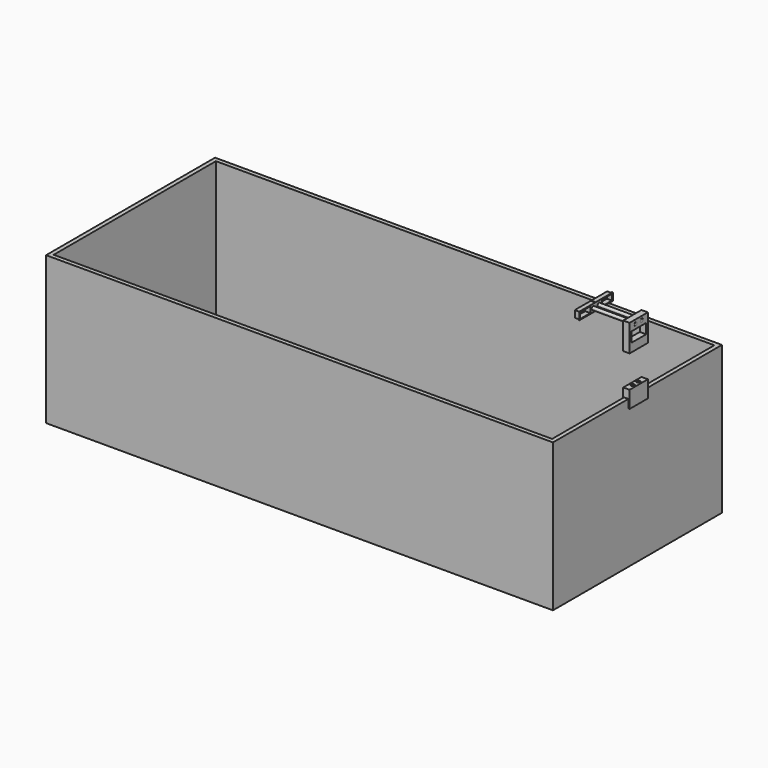
from build123d import *

# Parameters (mm, degrees)
F0_W          = 1.5
F0_H          = 1
F0_H_2        = 16
F0_R          = 4.25
F0_W_2        = 30
F0_H_3        = 14
F1_DEPTH      = 2
F2_DEPTH      = 10
F2_DEPTH_BACK = 2
F5_W          = 1200
F5_H          = 500
F5_W_2        = 1180
F5_H_2        = 480
F6_DEPTH      = 350
F8_W          = 10
F8_H          = 2
F8_W_2        = 1
F8_H_2        = 50
F8_R          = 4.25
F9_DEPTH      = 10
F8_W_3        = 11
F10_DEPTH     = 20
F12_DEPTH     = 15
F13_DEPTH     = 20
F14_W         = 54
F14_H         = 63.75
F14_R         = 4.25
F14_W_2       = 44
F14_H_2       = 23.75
F15_DEPTH     = 15
F16_W         = 110
F16_H         = 4
F19_R         = 4.25
F20_DEPTH     = 15


# Not quite as in the source:
# - a feature names something its author has since deleted; it is built from what else it names
# - the program builds the solid bodies; features that only make, move or delete a surface that nothing else refers to are left out


with BuildPart() as f1:
    # F0 (on Right) → F1 (new body)
    with BuildSketch(Plane.YZ):
        Polygon((-0.75, 9), (-49.5, 9), (-49.5, -9), (-0.75, -9), (-0.75, -8), (-13, -8), (-16, -8), (-48, -8), (-48, 8), (-16, 8), (-13, 8), (-0.75, 8), align=None)
        with Locations((0, 8.5)):
            Rectangle(F0_W, F0_H)
        Polygon((49.5, 9), (0.75, 9), (0.75, 8), (13, 8), (16, 8), (48, 8), (48, -8), (16, -8), (13, -8), (0.75, -8), (0.75, -9), (49.5, -9), align=None)
        with Locations((0, -8.5)):
            Rectangle(F0_W, F0_H)
        Rectangle(F0_W, F0_H_2)
        Polygon((13, 8), (0.75, 8), (0.75, -8), (13, -8), (16, -8), (48, -8), (48, 8), (16, 8), align=None)
        with Locations((8.75, 0)):
            Circle(F0_R, mode=Mode.SUBTRACT)
        with Locations((32, 0)):
            Rectangle(F0_W_2, F0_H_3, mode=Mode.SUBTRACT)
    extrude(amount=F1_DEPTH)

    # F0 (on Right) → F2 (join, two sides)
    with BuildSketch(Plane.YZ) as f2_sk:
        Polygon((-0.75, -8), (-0.75, 8), (-13, 8), (-16, 8), (-48, 8), (-48, -8), (-16, -8), (-13, -8), align=None)
        with Locations((-32, 0)):
            Rectangle(F0_W_2, F0_H_3, mode=Mode.SUBTRACT)
        with Locations((-8.75, 0)):
            Circle(F0_R, mode=Mode.SUBTRACT)
        Polygon((13, 8), (0.75, 8), (0.75, -8), (13, -8), (16, -8), (48, -8), (48, 8), (16, 8), align=None)
        with Locations((8.75, 0)):
            Circle(F0_R, mode=Mode.SUBTRACT)
        with Locations((32, 0)):
            Rectangle(F0_W_2, F0_H_3, mode=Mode.SUBTRACT)
    extrude(amount=-F2_DEPTH)
    extrude(f2_sk.sketch, amount=F2_DEPTH_BACK)


with BuildPart() as f6:
    # F5 (on offset) → F6 (new body)
    with BuildSketch(Plane.XY.offset(-500)):
        with Locations((-500, 0)):
            Rectangle(F5_W, F5_H)
        with Locations((-500, 0)):
            Rectangle(F5_W_2, F5_H_2, mode=Mode.SUBTRACT)
    extrude(amount=F6_DEPTH)


with BuildPart() as f9:
    # F8 (on face) → F9 (new body)
    with BuildSketch(Plane.XY.offset(-150)):
        Polygon((101, 27), (101, 25), (101, -25), (101, -27), (103, -27), (103, 27), align=None)
        Polygon((90, -25), (90, 25), (90, 27), (88, 27), (88, -27), (90, -27), align=None)
        with Locations((95, 26)):
            Rectangle(F8_W, F8_H)
        with Locations((100.5, 26)):
            Rectangle(F8_W_2, F8_H)
        with Locations((100.5, -26)):
            Rectangle(F8_W_2, F8_H)
        with Locations((95, -26)):
            Rectangle(F8_W, F8_H)
        with Locations((100.5, 0)):
            Rectangle(F8_W_2, F8_H_2)
        with Locations((95, 0)):
            Rectangle(F8_W, F8_H_2)
        with Locations((95.5, -8.75)):
            Circle(F8_R, mode=Mode.SUBTRACT)
        with Locations((95.5, 8.75)):
            Circle(F8_R, mode=Mode.SUBTRACT)
        with Locations((95.5, 8.75)):
            Circle(F8_R)
        with Locations((95.5, -8.75)):
            Circle(F8_R)
    extrude(amount=F9_DEPTH)

    # F8 (on face) → F10 (join)
    with BuildSketch(Plane.XY.offset(-150)):
        with Locations((95.5, 26)):
            Rectangle(F8_W_3, F8_H)
        Polygon((90, -25), (90, 25), (90, 27), (88, 27), (88, -27), (90, -27), align=None)
        Polygon((101, 27), (101, 25), (101, -25), (101, -27), (103, -27), (103, 27), align=None)
        with Locations((95.5, -26)):
            Rectangle(F8_W_3, F8_H)
        with Locations((95, 0)):
            Rectangle(F8_W, F8_H_2)
        with Locations((95.5, -8.75)):
            Circle(F8_R, mode=Mode.SUBTRACT)
        with Locations((95.5, 8.75)):
            Circle(F8_R, mode=Mode.SUBTRACT)
        with Locations((100.5, 0)):
            Rectangle(F8_W_2, F8_H_2)
    extrude(amount=F10_DEPTH)

    # F12 (add): a face of the model
    f12_faces = [f9.faces().sort_by_distance(p)[0] for p in [
        (95.5, 0, -130),
    ]]
    extrude(f12_faces, amount=-F12_DEPTH)

    # F8 (on face) → F13 (join)
    with BuildSketch(Plane.XY.offset(-150)):
        Polygon((90, -25), (90, 25), (90, 27), (88, 27), (88, -27), (90, -27), align=None)
        Polygon((101, 27), (101, 25), (101, -25), (101, -27), (103, -27), (103, 27), align=None)
    extrude(amount=-F13_DEPTH)


with BuildPart() as f15:
    # F14 (on face) → F15 (new body)
    with BuildSketch(Plane.YZ.offset(103)):
        with Locations((0, -22.375)):
            Rectangle(F14_W, F14_H)
        with Locations((-8.75, 0)):
            Circle(F14_R, mode=Mode.SUBTRACT)
        with Locations((0, -22.375)):
            Rectangle(F14_W_2, F14_H_2, mode=Mode.SUBTRACT)
        with Locations((8.75, 0)):
            Circle(F14_R, mode=Mode.SUBTRACT)
    extrude(amount=-F15_DEPTH)

    # F19 (on face) → F20 (cut)
    with BuildSketch(Plane(origin=(0, 0, -54.25), x_dir=(1, 0, 0), z_dir=(0, 0, -1))):
        with Locations((95.5, 8.75)):
            Circle(F19_R)
        with Locations((95.5, -8.75)):
            Circle(F19_R)
    extrude(amount=-F20_DEPTH, mode=Mode.SUBTRACT)


with BuildPart() as f17:
    # F16 (on Top) → F17 (revolve)
    with BuildSketch(Plane.XY):
        with Locations((48, -6.5)):
            Rectangle(F16_W, F16_H)
    revolve(axis=Axis((48, -8.5, 0), (1, 0, 0)))


with BuildPart() as f18:
    # F16 (on Top) → F18 (revolve)
    with BuildSketch(Plane.XY):
        with Locations((48, 6.5)):
            Rectangle(F16_W, F16_H)
    revolve(axis=Axis((48, 8.5, 0), (1, 0, 0)))


solid = Compound([f1.part, f6.part, f9.part, f15.part, f17.part, f18.part])
